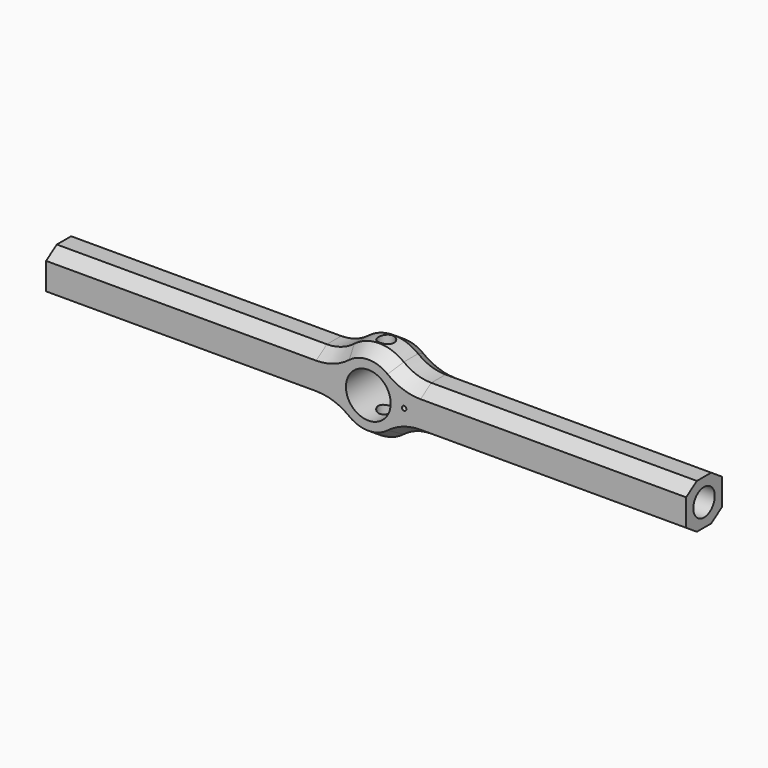
from build123d import *

# Parameters (mm, degrees)
F0_R          = 5
F0_R_2        = 0.5
F1_DEPTH      = 10
F2_R          = 3
F3_DEPTH      = 40
F4_R          = 1.75
F5_DEPTH      = 9.001
F5_DEPTH_BACK = 9.001
F6_R          = 10
F7_SIZE2      = 3
F7_SIZE       = 2
F7_2_SIZE2    = 3
F7_2_SIZE     = 2


# Not quite as in the source:
# - a pattern or mirror of a feature is missing from the dataset's text; its kind, count and spacing are read off the source's solid


with BuildPart() as f1:
    # F0 (on Front) → F1 (new body)
    with BuildSketch(Plane.XZ):
        with BuildLine():
            Line((71, 5), (7.4833147735, 5))
            ThreePointArc((7.4833147735, 5), (0, 9), (-7.4833147735, 5))
            Line((-7.4833147735, 5), (-72, 5))
            Line((-72, 5), (-72, -5))
            Line((-72, -5), (-7.4833147735, -5))
            ThreePointArc((-7.4833147735, -5), (0, -9), (7.4833147735, -5))
            Line((7.4833147735, -5), (71, -5))
            Line((71, -5), (71, 5))
        make_face()
        Circle(F0_R, mode=Mode.SUBTRACT)
        with Locations((8, 0)):
            Circle(F0_R_2, mode=Mode.SUBTRACT)
    extrude(amount=F1_DEPTH)

    # F2 (on face) → F3 (cut)
    with BuildSketch(Plane(origin=(-72, 0, 0), x_dir=(0, -1, 0), z_dir=(-1, 0, 0))):
        with Locations((5, 0)):
            Circle(F2_R)
    f3 = extrude(amount=-F3_DEPTH, mode=Mode.SUBTRACT)

    # F3_copies: F3 across plane
    add(f3.mirror(Plane(origin=(0, 0, 0), x_dir=(0, 0, 1), z_dir=(1, 0, 0))), mode=Mode.SUBTRACT)

    # F4 (on Top) → F5 (cut, two sides)
    with BuildSketch(Plane.XY) as f5_sk:
        with Locations((0, -5)):
            Circle(F4_R)
    extrude(amount=-F5_DEPTH, mode=Mode.SUBTRACT)
    extrude(f5_sk.sketch, amount=F5_DEPTH_BACK, mode=Mode.SUBTRACT)

    # F6
    f6_edges = [f1.edges().sort_by_distance(p)[0] for p in [
        (-7.483315, -5, 5),
        (7.483315, -5, 5),
        (7.483315, -5, -5),
        (-7.483315, -5, -5),
    ]]
    fillet(f6_edges, radius=F6_R)

    # F7
    f7_edges = [f1.edges().sort_by_distance(p)[0] for p in [
        (-41.830952, -10, 5),
        (-41.830952, -10, -5),
    ]]
    f7_side = f1.faces().sort_by_distance((41.330952, -10, -3.558716))[0]
    chamfer(f7_edges, length=F7_SIZE, length2=F7_SIZE2, reference=f7_side)

    # F7#2
    f7_2_edges = [f1.edges().sort_by_distance(p)[0] for p in [
        (-41.830952, 0, 5),
        (-41.830952, 0, -5),
    ]]
    f7_2_side = f1.faces().sort_by_distance((41.330952, 0, -3.558716))[0]
    chamfer(f7_2_edges, length=F7_2_SIZE, length2=F7_2_SIZE2, reference=f7_2_side)


solid = f1.part
